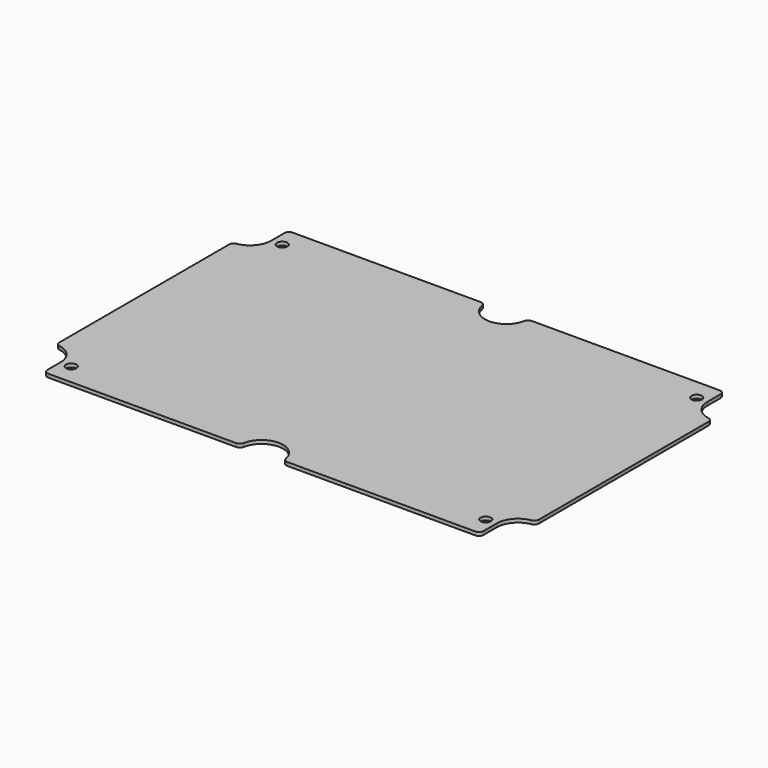
from build123d import *

# Parameters (mm, degrees)
F0_R     = 2.2500080016
F1_DEPTH = 1.524


# Not quite as in the source:
# - ends of sketch curves that miss each other by under 0.0002 mm in the source are joined


with BuildPart() as f1:
    # F0 (on Top) → F1 (new body)
    with BuildSketch(Plane.XY):
        with BuildLine():
            Line((-94.6519925541, -65.6767721), (-12.3569142118, -65.6767975))
            ThreePointArc((-12.3569142118, -65.6767975), (-11.0795804522, -65.2157564043), (-10.3911484863, -64.0452001887))
            ThreePointArc((-10.3911484863, -64.0452001887), (-1.1520076605, -56.3767915202), (8.0871293483, -64.0452047877))
            ThreePointArc((8.0871293483, -64.0452047877), (8.7758066433, -65.2159392609), (10.0535111494, -65.6767720058))
            Line((10.0535111494, -65.6767720058), (92.3479979541, -65.6767721))
            ThreePointArc((92.3479979541, -65.6767721), (93.7621995832, -65.0909958659), (94.3479937777, -63.6768016764))
            Line((94.3479937777, -63.6768016764), (94.3479937777, -56.4767913114))
            ThreePointArc((94.3479937777, -56.4767913114), (96.5686254579, -50.4091149721), (102.1813285767, -47.2082611927))
            ThreePointArc((102.1813285767, -47.2082611927), (103.3755112292, -46.5272203825), (103.8479739399, -45.2362255027))
            Line((103.8479739399, -45.2362255027), (103.8479739399, 47.6826559027))
            ThreePointArc((103.8479739399, 47.6826559027), (103.3755051193, 48.9736417855), (102.18132591, 49.6546758171))
            ThreePointArc((102.18132591, 49.6546758171), (96.5686275458, 52.8555266753), (94.3479937777, 58.9231963114))
            Line((94.3479937777, 58.9231963114), (94.3479937777, 66.1232066764))
            ThreePointArc((94.3479937777, 66.1232066764), (93.7622085633, 67.5374172856), (92.3479979541, 68.1232025))
            Line((92.3479979541, 68.1232025), (10.0528942103, 68.1232351277))
            ThreePointArc((10.0528942103, 68.1232351277), (8.7755585629, 67.662193921), (8.0871263436, 66.4916357508))
            ThreePointArc((8.0871263436, 66.4916357508), (-1.1520108709, 58.8232175176), (-10.3911530852, 66.4916297269))
            ThreePointArc((-10.3911530852, 66.4916297269), (-11.0795900575, 67.6621693766), (-12.3569142118, 68.1232025))
            Line((-12.3569142118, 68.1232025), (-94.6519925541, 68.1232025))
            ThreePointArc((-94.6519925541, 68.1232025), (-96.0662031633, 67.5374172856), (-96.6519883777, 66.1232066764))
            Line((-96.6519883777, 66.1232066764), (-96.6519883777, 58.9231963114))
            ThreePointArc((-96.6519883777, 58.9231963114), (-98.8726186915, 52.8555215887), (-104.4853190025, 49.6546668983))
            ThreePointArc((-104.4853190025, 49.6546668983), (-105.6795170362, 48.9736513496), (-106.1519939399, 47.6826559027))
            Line((-106.1519939399, 47.6826559027), (-106.1519939399, -45.2362255027))
            ThreePointArc((-106.1519939399, -45.2362255027), (-105.6795170362, -46.5272209496), (-104.4853212157, -47.2082495912))
            ThreePointArc((-104.4853212157, -47.2082495912), (-98.8726200579, -50.4091149721), (-96.6519883777, -56.4767913114))
            Line((-96.6519883777, -56.4767913114), (-96.6519883777, -63.6768016764))
            ThreePointArc((-96.6519883777, -63.6768016764), (-96.0661941832, -65.0909958659), (-94.6519925541, -65.6767721))
        make_face()
        with Locations((-91.9019855966, -56.526778507)):
            Circle(F0_R, mode=Mode.SUBTRACT)
        with Locations((89.5979909966, -56.526778507)):
            Circle(F0_R, mode=Mode.SUBTRACT)
        with Locations((-91.9019855966, 58.973208907)):
            Circle(F0_R, mode=Mode.SUBTRACT)
        with Locations((89.5979909966, 58.973208907)):
            Circle(F0_R, mode=Mode.SUBTRACT)
    extrude(amount=F1_DEPTH)


solid = f1.part
